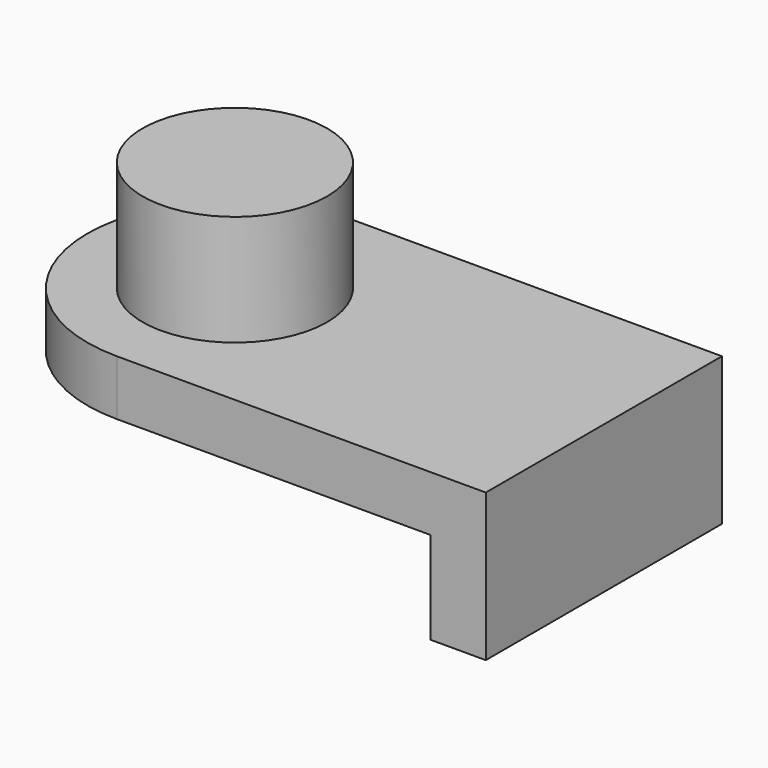
from build123d import *

# Parameters (mm, degrees)
F1_DEPTH = 101.6
F2_R     = 50.79999
F3_R     = 31.75
F4_DEPTH = 38.1


# Not quite as in the source:
# - a fillet or chamfer is up to 0.001 mm smaller than in the source, because OpenCascade refuses the exact size
# - the program builds the solid bodies; features that only make, move or delete a surface that nothing else refers to are left out


with BuildPart() as f1:
    # F0 (on Front) → F1 (new body)
    with BuildSketch(Plane.XZ):
        Polygon((-74.6155765653, -32.5891098499), (-74.6155765653, -51.6391098499), (84.1344234347, -51.6391098499), (84.1344234347, -79.0963023901), (84.1344234347, -83.3891098499), (103.1844234347, -83.3891098499), (103.1844234347, -32.5891098499), align=None)
    extrude(amount=F1_DEPTH)

    # F2 (radius 50.8 in the source; OpenCascade refuses exactly that, so slightly less here)
    f2_edges = [f1.edges().sort_by_distance(p)[0] for p in [
        (-74.615577, 0, -42.11411),
        (-74.615577, -101.6, -42.11411),
    ]]
    fillet(f2_edges, radius=F2_R)

    # F3 (on face) → F4 (join)
    with BuildSketch(Plane.XY.offset(-32.5891098499)):
        with Locations((-23.8155765653, -50.8)):
            Circle(F3_R)
    extrude(amount=F4_DEPTH)


solid = f1.part
